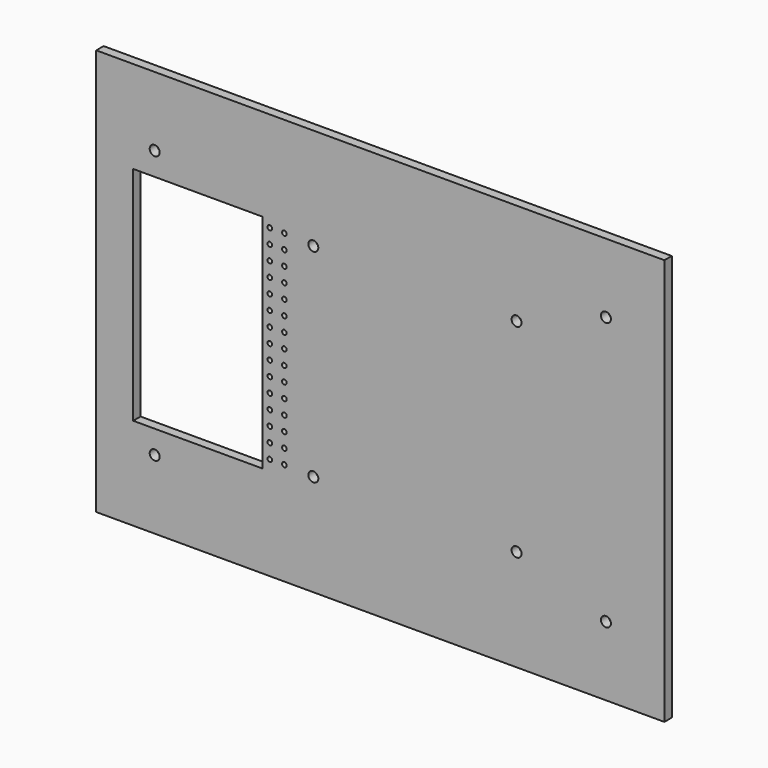
from build123d import *

# Parameters (mm, degrees)
F0_W     = 390.525
F0_H     = 279.4
F0_R     = 3.429
F0_R_2   = 1.6002
F0_W_2   = 88.9
F0_H_2   = 152.4
F1_DEPTH = 6.35


# Not quite as in the source:
# - a feature names something its author has since deleted; it is built from what else it names


with BuildPart() as f1:
    # F0 (on Front) → F1 (new body)
    with BuildSketch(Plane.XZ):
        with Locations((195.2625, -139.7)):
            Rectangle(F0_W, F0_H)
        with Locations((40.1828, -231.8004)):
            Circle(F0_R, mode=Mode.SUBTRACT)
        with Locations((149.225, -209.55)):
            Circle(F0_R, mode=Mode.SUBTRACT)
        with Locations((119.3038, -208.6864)):
            Circle(F0_R_2, mode=Mode.SUBTRACT)
        with Locations((119.3038, -198.6788)):
            Circle(F0_R_2, mode=Mode.SUBTRACT)
        with Locations((129.3114, -208.6864)):
            Circle(F0_R_2, mode=Mode.SUBTRACT)
        with Locations((129.3114, -198.6788)):
            Circle(F0_R_2, mode=Mode.SUBTRACT)
        with Locations((119.3038, -188.6712)):
            Circle(F0_R_2, mode=Mode.SUBTRACT)
        with Locations((119.3038, -178.6636)):
            Circle(F0_R_2, mode=Mode.SUBTRACT)
        with Locations((129.3114, -188.6712)):
            Circle(F0_R_2, mode=Mode.SUBTRACT)
        with Locations((129.3114, -178.6636)):
            Circle(F0_R_2, mode=Mode.SUBTRACT)
        with Locations((119.3038, -168.656)):
            Circle(F0_R_2, mode=Mode.SUBTRACT)
        with Locations((119.3038, -158.6484)):
            Circle(F0_R_2, mode=Mode.SUBTRACT)
        with Locations((129.3114, -168.656)):
            Circle(F0_R_2, mode=Mode.SUBTRACT)
        with Locations((129.3114, -158.6484)):
            Circle(F0_R_2, mode=Mode.SUBTRACT)
        with Locations((119.3038, -148.6408)):
            Circle(F0_R_2, mode=Mode.SUBTRACT)
        with Locations((129.3114, -148.6408)):
            Circle(F0_R_2, mode=Mode.SUBTRACT)
        with Locations((288.925, -209.55)):
            Circle(F0_R, mode=Mode.SUBTRACT)
        with Locations((350.3422, -231.8004)):
            Circle(F0_R, mode=Mode.SUBTRACT)
        with Locations((69.85, -139.7)):
            Rectangle(F0_W_2, F0_H_2, mode=Mode.SUBTRACT)
        with Locations((119.3038, -138.6332)):
            Circle(F0_R_2, mode=Mode.SUBTRACT)
        with Locations((119.3038, -128.6256)):
            Circle(F0_R_2, mode=Mode.SUBTRACT)
        with Locations((129.3114, -138.6332)):
            Circle(F0_R_2, mode=Mode.SUBTRACT)
        with Locations((129.3114, -128.6256)):
            Circle(F0_R_2, mode=Mode.SUBTRACT)
        with Locations((119.3038, -118.618)):
            Circle(F0_R_2, mode=Mode.SUBTRACT)
        with Locations((119.3038, -108.6104)):
            Circle(F0_R_2, mode=Mode.SUBTRACT)
        with Locations((129.3114, -118.618)):
            Circle(F0_R_2, mode=Mode.SUBTRACT)
        with Locations((129.3114, -108.6104)):
            Circle(F0_R_2, mode=Mode.SUBTRACT)
        with Locations((119.3038, -98.6028)):
            Circle(F0_R_2, mode=Mode.SUBTRACT)
        with Locations((119.3038, -88.5952)):
            Circle(F0_R_2, mode=Mode.SUBTRACT)
        with Locations((129.3114, -98.6028)):
            Circle(F0_R_2, mode=Mode.SUBTRACT)
        with Locations((129.3114, -88.5952)):
            Circle(F0_R_2, mode=Mode.SUBTRACT)
        with Locations((119.3038, -78.5876)):
            Circle(F0_R_2, mode=Mode.SUBTRACT)
        with Locations((129.3114, -78.5876)):
            Circle(F0_R_2, mode=Mode.SUBTRACT)
        with Locations((40.1701, -47.5869)):
            Circle(F0_R, mode=Mode.SUBTRACT)
        with Locations((119.3038, -68.58)):
            Circle(F0_R_2, mode=Mode.SUBTRACT)
        with Locations((129.3114, -68.58)):
            Circle(F0_R_2, mode=Mode.SUBTRACT)
        with Locations((149.225, -69.85)):
            Circle(F0_R, mode=Mode.SUBTRACT)
        with Locations((288.925, -69.85)):
            Circle(F0_R, mode=Mode.SUBTRACT)
        with Locations((350.3422, -47.5996)):
            Circle(F0_R, mode=Mode.SUBTRACT)
    extrude(amount=F1_DEPTH)


solid = f1.part
